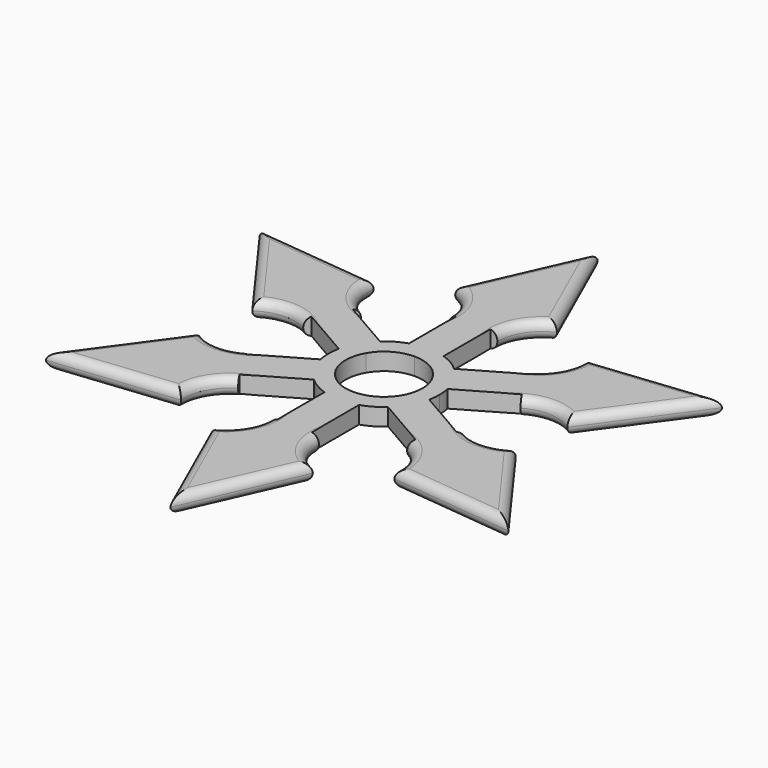
from build123d import *

# Parameters (mm, degrees)
F1_DEPTH     = 5
F2_DEPTH     = 5
F3_T1_DEPTH  = 48.744289009
F3_T3_DEPTH  = 48.744289009
F3_T5_DEPTH  = 48.744289009
F3_T7_DEPTH  = 48.744289009
F3_T9_DEPTH  = 48.744289009
F3_T11_DEPTH = 48.744289009
F3_T13_DEPTH = 48.744289009
F3_T15_DEPTH = 48.744289009
F3_T17_DEPTH = 48.744289009
F3_T19_DEPTH = 48.744289009
F3_T21_DEPTH = 48.744289009
F3_T23_DEPTH = 48.744289009
F3_T26_ANGLE = 121.141520227
F3_T28_ANGLE = 121.141520227
F3_T30_ANGLE = 121.141520227
F3_T32_ANGLE = 121.141520227
F3_T34_ANGLE = 121.141520227
F3_T36_ANGLE = 121.141520227
F3_T38_ANGLE = 121.141520227
F3_T40_ANGLE = 121.141520227
F3_T42_ANGLE = 121.141520227
F3_T44_ANGLE = 121.141520227
F3_T46_ANGLE = 121.141520227
F3_T48_ANGLE = 121.141520227
F3_T50_ANGLE = 121.141520227
F3_T52_ANGLE = 121.141520227
F3_T54_ANGLE = 121.141520227
F3_T56_ANGLE = 121.141520227
F3_T58_ANGLE = 121.141520227
F3_T60_ANGLE = 121.141520227
F3_T62_ANGLE = 121.141520227
F3_T64_ANGLE = 121.141520227
F3_T66_ANGLE = 121.141520227
F3_T68_ANGLE = 121.141520227
F3_T70_ANGLE = 121.141520227
F3_T72_ANGLE = 121.141520227


# Not quite as in the source:
# - a fillet or chamfer that OpenCascade refuses, or shapes differently, is made with other operations: its cross-section is extruded or revolved along the edge and cut away or added


with BuildPart() as f1:
    # F0 (on Top) → F1 (new body)
    with BuildSketch(Plane.XY):
        with BuildLine():
            Line((-27.9760162852, 16.1519605331), (-13.9430090009, 8.05))
            ThreePointArc((-13.9430090009, 8.05), (-12.5038298049, 10.142200955), (-10.7535844208, 11.982087552))
            Line((-10.7535844208, 11.982087552), (-25.4760162852, 20.482087552))
            Line((-25.4760162852, 20.482087552), (-27.9760162852, 16.1519605331))
        make_face()
        with BuildLine():
            ThreePointArc((-15.7535844208, 3.3218335142), (-15.0353185797, 5.7575337781), (-13.9430090009, 8.05))
            Line((-13.9430090009, 8.05), (-27.9760162852, 16.1519605331))
            Line((-27.9760162852, 16.1519605331), (-30.4760162852, 11.8218335142))
            Line((-30.4760162852, 11.8218335142), (-15.7535844208, 3.3218335142))
        make_face()
        with BuildLine():
            ThreePointArc((-9.612881982, -5.55), (-11.1, 0), (-9.612881982, 5.55))
            Line((-9.612881982, 5.55), (-13.9430090009, 8.05))
            ThreePointArc((-13.9430090009, 8.05), (-15.0353185797, 5.7575337781), (-15.7535844208, 3.3218335142))
            ThreePointArc((-15.7535844208, 3.3218335142), (-16.1, 0), (-15.7535844208, -3.3218335142))
            ThreePointArc((-15.7535844208, -3.3218335142), (-15.0353185797, -5.7575337781), (-13.9430090009, -8.05))
            Line((-13.9430090009, -8.05), (-9.612881982, -5.55))
        make_face()
        with BuildLine():
            ThreePointArc((-9.612881982, 5.55), (-5.55, 9.612881982), (0, 11.1))
            Line((0, 11.1), (0, 16.1))
            ThreePointArc((0, 16.1), (-2.5314887749, 15.8997347331), (-5, 15.3039210662))
            ThreePointArc((-5, 15.3039210662), (-8.05, 13.9430090009), (-10.7535844208, 11.982087552))
            ThreePointArc((-10.7535844208, 11.982087552), (-12.5038298049, 10.142200955), (-13.9430090009, 8.05))
            Line((-13.9430090009, 8.05), (-9.612881982, 5.55))
        make_face()
        with BuildLine():
            ThreePointArc((0, 11.1), (5.55, 9.612881982), (9.612881982, 5.55))
            Line((9.612881982, 5.55), (13.9430090009, 8.05))
            ThreePointArc((13.9430090009, 8.05), (12.5038298049, 10.142200955), (10.7535844208, 11.982087552))
            ThreePointArc((10.7535844208, 11.982087552), (8.05, 13.9430090009), (5, 15.3039210662))
            ThreePointArc((5, 15.3039210662), (2.5314887749, 15.8997347331), (0, 16.1))
            Line((0, 16.1), (0, 11.1))
        make_face()
        with BuildLine():
            ThreePointArc((9.612881982, 5.55), (10.7217766718, 2.8728914006), (11.1, 0))
            ThreePointArc((11.1, 0), (10.7217766718, -2.8728914006), (9.612881982, -5.55))
            Line((9.612881982, -5.55), (13.9430090009, -8.05))
            ThreePointArc((13.9430090009, -8.05), (15.0353185797, -5.7575337781), (15.7535844208, -3.3218335142))
            ThreePointArc((15.7535844208, -3.3218335142), (16.0131619172, -1.6699237744), (16.1, 0))
            ThreePointArc((16.1, 0), (16.0131619172, 1.6699237744), (15.7535844208, 3.3218335142))
            ThreePointArc((15.7535844208, 3.3218335142), (15.0353185797, 5.7575337781), (13.9430090009, 8.05))
            Line((13.9430090009, 8.05), (9.612881982, 5.55))
        make_face()
        with BuildLine():
            Line((13.9430090009, -8.05), (9.612881982, -5.55))
            ThreePointArc((9.612881982, -5.55), (5.55, -9.612881982), (0, -11.1))
            Line((0, -11.1), (0, -16.1))
            ThreePointArc((0, -16.1), (2.5314887749, -15.8997347331), (5, -15.3039210662))
            ThreePointArc((5, -15.3039210662), (8.05, -13.9430090009), (10.7535844208, -11.982087552))
            ThreePointArc((10.7535844208, -11.982087552), (12.5038298049, -10.142200955), (13.9430090009, -8.05))
        make_face()
        with BuildLine():
            Line((0, -16.1), (0, -11.1))
            ThreePointArc((0, -11.1), (-5.55, -9.612881982), (-9.612881982, -5.55))
            Line((-9.612881982, -5.55), (-13.9430090009, -8.05))
            ThreePointArc((-13.9430090009, -8.05), (-12.5038298049, -10.142200955), (-10.7535844208, -11.982087552))
            ThreePointArc((-10.7535844208, -11.982087552), (-8.05, -13.9430090009), (-5, -15.3039210662))
            ThreePointArc((-5, -15.3039210662), (-2.5314887749, -15.8997347331), (0, -16.1))
        make_face()
        with BuildLine():
            ThreePointArc((-10.7535844208, -11.982087552), (-12.5038298049, -10.142200955), (-13.9430090009, -8.05))
            Line((-13.9430090009, -8.05), (-27.9760162852, -16.1519605331))
            Line((-27.9760162852, -16.1519605331), (-25.4760162852, -20.482087552))
            Line((-25.4760162852, -20.482087552), (-10.7535844208, -11.982087552))
        make_face()
        with BuildLine():
            Line((-27.9760162852, -16.1519605331), (-13.9430090009, -8.05))
            ThreePointArc((-13.9430090009, -8.05), (-15.0353185797, -5.7575337781), (-15.7535844208, -3.3218335142))
            Line((-15.7535844208, -3.3218335142), (-30.4760162852, -11.8218335142))
            Line((-30.4760162852, -11.8218335142), (-27.9760162852, -16.1519605331))
        make_face()
        with BuildLine():
            ThreePointArc((10.7535844208, 11.982087552), (12.5038298049, 10.142200955), (13.9430090009, 8.05))
            Line((13.9430090009, 8.05), (27.9760162852, 16.1519605331))
            Line((27.9760162852, 16.1519605331), (25.4760162852, 20.482087552))
            Line((25.4760162852, 20.482087552), (10.7535844208, 11.982087552))
        make_face()
        with BuildLine():
            Line((27.9760162852, 16.1519605331), (13.9430090009, 8.05))
            ThreePointArc((13.9430090009, 8.05), (15.0353185797, 5.7575337781), (15.7535844208, 3.3218335142))
            Line((15.7535844208, 3.3218335142), (30.4760162852, 11.8218335142))
            Line((30.4760162852, 11.8218335142), (27.9760162852, 16.1519605331))
        make_face()
        with BuildLine():
            Line((0, 32.3039210662), (0, 16.1))
            ThreePointArc((0, 16.1), (2.5314887749, 15.8997347331), (5, 15.3039210662))
            Line((5, 15.3039210662), (5, 32.3039210662))
            Line((5, 32.3039210662), (0, 32.3039210662))
        make_face()
        with BuildLine():
            ThreePointArc((-5, 15.3039210662), (-2.5314887749, 15.8997347331), (0, 16.1))
            Line((0, 16.1), (0, 32.3039210662))
            Line((0, 32.3039210662), (-5, 32.3039210662))
            Line((-5, 32.3039210662), (-5, 15.3039210662))
        make_face()
        with BuildLine():
            ThreePointArc((15.7535844208, -3.3218335142), (15.0353185797, -5.7575337781), (13.9430090009, -8.05))
            Line((13.9430090009, -8.05), (27.9760162852, -16.1519605331))
            Line((27.9760162852, -16.1519605331), (30.4760162852, -11.8218335142))
            Line((30.4760162852, -11.8218335142), (15.7535844208, -3.3218335142))
        make_face()
        with BuildLine():
            Line((27.9760162852, -16.1519605331), (13.9430090009, -8.05))
            ThreePointArc((13.9430090009, -8.05), (12.5038298049, -10.142200955), (10.7535844208, -11.982087552))
            Line((10.7535844208, -11.982087552), (25.4760162852, -20.482087552))
            Line((25.4760162852, -20.482087552), (27.9760162852, -16.1519605331))
        make_face()
        with BuildLine():
            ThreePointArc((5, -15.3039210662), (2.5314887749, -15.8997347331), (0, -16.1))
            Line((0, -16.1), (0, -32.3039210662))
            Line((0, -32.3039210662), (5, -32.3039210662))
            Line((5, -32.3039210662), (5, -15.3039210662))
        make_face()
        with BuildLine():
            Line((0, -32.3039210662), (0, -16.1))
            ThreePointArc((0, -16.1), (-2.5314887749, -15.8997347331), (-5, -15.3039210662))
            Line((-5, -15.3039210662), (-5, -32.3039210662))
            Line((-5, -32.3039210662), (0, -32.3039210662))
        make_face()
    extrude(amount=F1_DEPTH)

    # F0 (on Top) → F2 (join)
    with BuildSketch(Plane.XY):
        with BuildLine():
            Line((-66.9471594555, 38.6519605331), (-27.9760162852, 16.1519605331))
            Line((-27.9760162852, 16.1519605331), (-25.4760162852, 20.482087552))
            Line((-25.4760162852, 20.482087552), (-24.4760162852, 22.2141383596))
            ThreePointArc((-24.4760162852, 22.2141383596), (-29.5610324314, 27.5743840984), (-30.9039085144, 34.8398026971))
            Line((-30.9039085144, 34.8398026971), (-66.9471594555, 38.6519605331))
        make_face()
        with BuildLine():
            Line((-30.4760162852, 11.8218335142), (-27.9760162852, 16.1519605331))
            Line((-27.9760162852, 16.1519605331), (-66.9471594555, 38.6519605331))
            Line((-66.9471594555, 38.6519605331), (-45.6241084557, 9.3436685012))
            ThreePointArc((-45.6241084557, 9.3436685012), (-38.6606333386, 11.8134129985), (-31.4760162852, 10.0897827066))
            Line((-31.4760162852, 10.0897827066), (-30.4760162852, 11.8218335142))
        make_face()
        with BuildLine():
            Line((-5, 32.3039210662), (0, 32.3039210662))
            Line((0, 32.3039210662), (0, 77.3039210662))
            Line((0, 77.3039210662), (-14.7201999413, 44.1834711982))
            ThreePointArc((-14.7201999413, 44.1834711982), (-9.0996009072, 39.3877970969), (-7, 32.3039210662))
            Line((-7, 32.3039210662), (-5, 32.3039210662))
        make_face()
        with BuildLine():
            Line((0, 77.3039210662), (0, 32.3039210662))
            Line((0, 32.3039210662), (5, 32.3039210662))
            Line((5, 32.3039210662), (7, 32.3039210662))
            ThreePointArc((7, 32.3039210662), (9.0996009072, 39.3877970969), (14.7201999413, 44.1834711982))
            Line((14.7201999413, 44.1834711982), (0, 77.3039210662))
        make_face()
        with BuildLine():
            Line((25.4760162852, 20.482087552), (27.9760162852, 16.1519605331))
            Line((27.9760162852, 16.1519605331), (66.9471594555, 38.6519605331))
            Line((66.9471594555, 38.6519605331), (30.9039085144, 34.8398026971))
            ThreePointArc((30.9039085144, 34.8398026971), (29.5610324314, 27.5743840984), (24.4760162852, 22.2141383596))
            Line((24.4760162852, 22.2141383596), (25.4760162852, 20.482087552))
        make_face()
        with BuildLine():
            Line((66.9471594555, 38.6519605331), (27.9760162852, 16.1519605331))
            Line((27.9760162852, 16.1519605331), (30.4760162852, 11.8218335142))
            Line((30.4760162852, 11.8218335142), (31.4760162852, 10.0897827066))
            ThreePointArc((31.4760162852, 10.0897827066), (38.6606333386, 11.8134129985), (45.6241084557, 9.3436685012))
            Line((45.6241084557, 9.3436685012), (66.9471594555, 38.6519605331))
        make_face()
        with BuildLine():
            Line((30.4760162852, -11.8218335142), (27.9760162852, -16.1519605331))
            Line((27.9760162852, -16.1519605331), (66.9471594555, -38.6519605331))
            Line((66.9471594555, -38.6519605331), (45.6241084557, -9.3436685012))
            ThreePointArc((45.6241084557, -9.3436685012), (38.6606333386, -11.8134129985), (31.4760162852, -10.0897827066))
            Line((31.4760162852, -10.0897827066), (30.4760162852, -11.8218335142))
        make_face()
        with BuildLine():
            Line((66.9471594555, -38.6519605331), (27.9760162852, -16.1519605331))
            Line((27.9760162852, -16.1519605331), (25.4760162852, -20.482087552))
            Line((25.4760162852, -20.482087552), (24.4760162852, -22.2141383596))
            ThreePointArc((24.4760162852, -22.2141383596), (29.5610324314, -27.5743840984), (30.9039085144, -34.8398026971))
            Line((30.9039085144, -34.8398026971), (66.9471594555, -38.6519605331))
        make_face()
        with BuildLine():
            Line((5, -32.3039210662), (0, -32.3039210662))
            Line((0, -32.3039210662), (0, -77.3039210662))
            Line((0, -77.3039210662), (14.7201999413, -44.1834711982))
            ThreePointArc((14.7201999413, -44.1834711982), (9.0996009072, -39.3877970969), (7, -32.3039210662))
            Line((7, -32.3039210662), (5, -32.3039210662))
        make_face()
        with BuildLine():
            Line((0, -77.3039210662), (0, -32.3039210662))
            Line((0, -32.3039210662), (-5, -32.3039210662))
            Line((-5, -32.3039210662), (-7, -32.3039210662))
            ThreePointArc((-7, -32.3039210662), (-9.0996009072, -39.3877970969), (-14.7201999413, -44.1834711982))
            Line((-14.7201999413, -44.1834711982), (0, -77.3039210662))
        make_face()
        with BuildLine():
            Line((-25.4760162852, -20.482087552), (-27.9760162852, -16.1519605331))
            Line((-27.9760162852, -16.1519605331), (-66.9471594555, -38.6519605331))
            Line((-66.9471594555, -38.6519605331), (-30.9039085144, -34.8398026971))
            ThreePointArc((-30.9039085144, -34.8398026971), (-29.5610324314, -27.5743840984), (-24.4760162852, -22.2141383596))
            Line((-24.4760162852, -22.2141383596), (-25.4760162852, -20.482087552))
        make_face()
        with BuildLine():
            Line((-66.9471594555, -38.6519605331), (-27.9760162852, -16.1519605331))
            Line((-27.9760162852, -16.1519605331), (-30.4760162852, -11.8218335142))
            Line((-30.4760162852, -11.8218335142), (-31.4760162852, -10.0897827066))
            ThreePointArc((-31.4760162852, -10.0897827066), (-38.6606333386, -11.8134129985), (-45.6241084557, -9.3436685012))
            Line((-45.6241084557, -9.3436685012), (-66.9471594555, -38.6519605331))
        make_face()
    extrude(amount=F2_DEPTH)

    # F3: fillet of radius 2.5 on 48 edges, made by hand

    # F3_s2 → F3_t1 (cut)
    with BuildSketch(Plane(origin=(-76.4647193498, -8.0873831144, 0), x_dir=(0, 0, 1), z_dir=(0.9944532484, 0.1051795453, 0))):
        with BuildLine():
            ThreePointArc((5, 28.8960959217), (4.267766953, 30.6638628747), (2.5, 31.3960959217))
            Line((2.5, 31.3960959217), (5, 31.3960959217))
            Line((5, 31.3960959217), (5, 28.8960959217))
        make_face()
        with BuildLine():
            ThreePointArc((0, 28.8960959217), (0.732233047, 30.6638628747), (2.5, 31.3960959217))
            Line((2.5, 31.3960959217), (0, 31.3960959217))
            Line((0, 31.3960959217), (0, 28.8960959217))
        make_face()
    extrude(amount=F3_T1_DEPTH, mode=Mode.SUBTRACT)

    # F3_s4 → F3_t3 (cut)
    with BuildSketch(Plane(origin=(-16.5592531229, -22.760505819, 0), x_dir=(0, 0, 1), z_dir=(-0.5883147824, -0.8086320034, 0))):
        with BuildLine():
            ThreePointArc((5, 28.8960959217), (4.267766953, 30.6638628747), (2.5, 31.3960959217))
            Line((2.5, 31.3960959217), (5, 31.3960959217))
            Line((5, 31.3960959217), (5, 28.8960959217))
        make_face()
        with BuildLine():
            ThreePointArc((0, 28.8960959217), (0.732233047, 30.6638628747), (2.5, 31.3960959217))
            Line((2.5, 31.3960959217), (0, 31.3960959217))
            Line((0, 31.3960959217), (0, 28.8960959217))
        make_face()
    extrude(amount=F3_T3_DEPTH, mode=Mode.SUBTRACT)

    # F3_s6 → F3_t5 (cut)
    with BuildSketch(Plane(origin=(11.4315496807, -25.7209867816, 0), x_dir=(0, 0, 1), z_dir=(0.4061384661, -0.9138115486, 0))):
        with BuildLine():
            ThreePointArc((5, 28.8960959217), (4.267766953, 30.6638628747), (2.5, 31.3960959217))
            Line((2.5, 31.3960959217), (5, 31.3960959217))
            Line((5, 31.3960959217), (5, 28.8960959217))
        make_face()
        with BuildLine():
            ThreePointArc((0, 28.8960959217), (0.732233047, 30.6638628747), (2.5, 31.3960959217))
            Line((2.5, 31.3960959217), (0, 31.3960959217))
            Line((0, 31.3960959217), (0, 28.8960959217))
        make_face()
    extrude(amount=F3_T5_DEPTH, mode=Mode.SUBTRACT)

    # F3_s8 → F3_t7 (cut)
    with BuildSketch(Plane(origin=(-31.2284804477, -70.2640810073, 0), x_dir=(0, 0, 1), z_dir=(0.4061384661, 0.9138115486, 0))):
        with BuildLine():
            ThreePointArc((5, 28.8960959217), (4.267766953, 30.6638628747), (2.5, 31.3960959217))
            Line((2.5, 31.3960959217), (5, 31.3960959217))
            Line((5, 31.3960959217), (5, 28.8960959217))
        make_face()
        with BuildLine():
            ThreePointArc((0, 28.8960959217), (0.732233047, 30.6638628747), (2.5, 31.3960959217))
            Line((2.5, 31.3960959217), (0, 31.3960959217))
            Line((0, 31.3960959217), (0, 28.8960959217))
        make_face()
    extrude(amount=F3_T7_DEPTH, mode=Mode.SUBTRACT)

    # F3_s10 → F3_t9 (cut)
    with BuildSketch(Plane(origin=(45.2362389021, -62.176697893, 0), x_dir=(0, 0, 1), z_dir=(-0.5883147824, 0.8086320034, 0))):
        with BuildLine():
            ThreePointArc((5, 28.8960959217), (4.267766953, 30.6638628747), (2.5, 31.3960959217))
            Line((2.5, 31.3960959217), (5, 31.3960959217))
            Line((5, 31.3960959217), (5, 28.8960959217))
        make_face()
        with BuildLine():
            ThreePointArc((0, 28.8960959217), (0.732233047, 30.6638628747), (2.5, 31.3960959217))
            Line((2.5, 31.3960959217), (0, 31.3960959217))
            Line((0, 31.3960959217), (0, 28.8960959217))
        make_face()
    extrude(amount=F3_T9_DEPTH, mode=Mode.SUBTRACT)

    # F3_s12 → F3_t11 (cut)
    with BuildSketch(Plane(origin=(27.9908028037, -2.9604809627, 0), x_dir=(0, 0, 1), z_dir=(0.9944532484, -0.1051795453, 0))):
        with BuildLine():
            ThreePointArc((5, 28.8960959217), (4.267766953, 30.6638628747), (2.5, 31.3960959217))
            Line((2.5, 31.3960959217), (5, 31.3960959217))
            Line((5, 31.3960959217), (5, 28.8960959217))
        make_face()
        with BuildLine():
            ThreePointArc((0, 28.8960959217), (0.732233047, 30.6638628747), (2.5, 31.3960959217))
            Line((2.5, 31.3960959217), (0, 31.3960959217))
            Line((0, 31.3960959217), (0, 28.8960959217))
        make_face()
    extrude(amount=F3_T11_DEPTH, mode=Mode.SUBTRACT)

    # F3_s14 → F3_t13 (cut)
    with BuildSketch(Plane(origin=(76.4647193498, 8.0873831144, 0), x_dir=(0, 0, 1), z_dir=(-0.9944532484, -0.1051795453, 0))):
        with BuildLine():
            ThreePointArc((5, 28.8960959217), (4.267766953, 30.6638628747), (2.5, 31.3960959217))
            Line((2.5, 31.3960959217), (5, 31.3960959217))
            Line((5, 31.3960959217), (5, 28.8960959217))
        make_face()
        with BuildLine():
            ThreePointArc((0, 28.8960959217), (0.732233047, 30.6638628747), (2.5, 31.3960959217))
            Line((2.5, 31.3960959217), (0, 31.3960959217))
            Line((0, 31.3960959217), (0, 28.8960959217))
        make_face()
    extrude(amount=F3_T13_DEPTH, mode=Mode.SUBTRACT)

    # F3_s16 → F3_t15 (cut)
    with BuildSketch(Plane(origin=(16.5592531229, 22.760505819, 0), x_dir=(0, 0, 1), z_dir=(0.5883147824, 0.8086320034, 0))):
        with BuildLine():
            ThreePointArc((5, 28.8960959217), (4.267766953, 30.6638628747), (2.5, 31.3960959217))
            Line((2.5, 31.3960959217), (5, 31.3960959217))
            Line((5, 31.3960959217), (5, 28.8960959217))
        make_face()
        with BuildLine():
            ThreePointArc((0, 28.8960959217), (0.732233047, 30.6638628747), (2.5, 31.3960959217))
            Line((2.5, 31.3960959217), (0, 31.3960959217))
            Line((0, 31.3960959217), (0, 28.8960959217))
        make_face()
    extrude(amount=F3_T15_DEPTH, mode=Mode.SUBTRACT)

    # F3_s18 → F3_t17 (cut)
    with BuildSketch(Plane(origin=(-27.9908028037, 2.9604809627, 0), x_dir=(0, 0, 1), z_dir=(-0.9944532484, 0.1051795453, 0))):
        with BuildLine():
            ThreePointArc((2.5, 31.3960959217), (4.267766953, 30.6638628747), (5, 28.8960959217))
            Line((5, 28.8960959217), (5, 31.3960959217))
            Line((5, 31.3960959217), (2.5, 31.3960959217))
        make_face()
        with BuildLine():
            ThreePointArc((2.5, 31.3960959217), (0.732233047, 30.6638628747), (0, 28.8960959217))
            Line((0, 28.8960959217), (0, 31.3960959217))
            Line((0, 31.3960959217), (2.5, 31.3960959217))
        make_face()
    extrude(amount=F3_T17_DEPTH, mode=Mode.SUBTRACT)

    # F3_s20 → F3_t19 (cut)
    with BuildSketch(Plane(origin=(-45.2362389021, 62.176697893, 0), x_dir=(0, 0, 1), z_dir=(0.5883147824, -0.8086320034, 0))):
        with BuildLine():
            ThreePointArc((2.5, 31.3960959217), (4.267766953, 30.6638628747), (5, 28.8960959217))
            Line((5, 28.8960959217), (5, 31.3960959217))
            Line((5, 31.3960959217), (2.5, 31.3960959217))
        make_face()
        with BuildLine():
            ThreePointArc((2.5, 31.3960959217), (0.732233047, 30.6638628747), (0, 28.8960959217))
            Line((0, 28.8960959217), (0, 31.3960959217))
            Line((0, 31.3960959217), (2.5, 31.3960959217))
        make_face()
    extrude(amount=F3_T19_DEPTH, mode=Mode.SUBTRACT)

    # F3_s22 → F3_t21 (cut)
    with BuildSketch(Plane(origin=(31.2284804477, 70.2640810073, 0), x_dir=(0, 0, 1), z_dir=(-0.4061384661, -0.9138115486, 0))):
        with BuildLine():
            ThreePointArc((5, 28.8960959217), (4.267766953, 30.6638628747), (2.5, 31.3960959217))
            Line((2.5, 31.3960959217), (5, 31.3960959217))
            Line((5, 31.3960959217), (5, 28.8960959217))
        make_face()
        with BuildLine():
            ThreePointArc((0, 28.8960959217), (0.732233047, 30.6638628747), (2.5, 31.3960959217))
            Line((2.5, 31.3960959217), (0, 31.3960959217))
            Line((0, 31.3960959217), (0, 28.8960959217))
        make_face()
    extrude(amount=F3_T21_DEPTH, mode=Mode.SUBTRACT)

    # F3_s24 → F3_t23 (cut)
    with BuildSketch(Plane(origin=(-11.4315496807, 25.7209867816, 0), x_dir=(0, 0, 1), z_dir=(-0.4061384661, 0.9138115486, 0))):
        with BuildLine():
            ThreePointArc((5, 28.8960959217), (4.267766953, 30.6638628747), (2.5, 31.3960959217))
            Line((2.5, 31.3960959217), (5, 31.3960959217))
            Line((5, 31.3960959217), (5, 28.8960959217))
        make_face()
        with BuildLine():
            ThreePointArc((0, 28.8960959217), (0.732233047, 30.6638628747), (2.5, 31.3960959217))
            Line((2.5, 31.3960959217), (0, 31.3960959217))
            Line((0, 31.3960959217), (0, 28.8960959217))
        make_face()
    extrude(amount=F3_T23_DEPTH, mode=Mode.SUBTRACT)

    # F3_s25 → F3_t26 (revolve, cut)
    with BuildSketch(Plane(origin=(19.3716122948, -0.8281673611, 0), x_dir=(0, 0, 1), z_dir=(-0.9990874013, 0.0427125819, 0))):
        with BuildLine():
            ThreePointArc((0, -17.1741196082), (0.732233047, -18.9418865612), (2.5, -19.6741196082))
            Line((2.5, -19.6741196082), (0, -19.6741196082))
            Line((0, -19.6741196082), (0, -17.1741196082))
        make_face()
    revolve(axis=Axis((17.9760162852, -33.4724686088, 0), (0, 0, -1)), revolution_arc=F3_T26_ANGLE, mode=Mode.SUBTRACT)

    # F3_s27 → F3_t28 (revolve, cut)
    with BuildSketch(Plane(origin=(19.3716122948, -0.8281673611, 0), x_dir=(0, 0, 1), z_dir=(-0.9990874013, 0.0427125819, 0))):
        with BuildLine():
            ThreePointArc((5, -17.1741196082), (4.267766953, -18.9418865612), (2.5, -19.6741196082))
            Line((2.5, -19.6741196082), (5, -19.6741196082))
            Line((5, -19.6741196082), (5, -17.1741196082))
        make_face()
    revolve(axis=Axis((17.9760162852, -33.4724686088, 5), (0, 0, -1)), revolution_arc=F3_T28_ANGLE, mode=Mode.SUBTRACT)

    # F3_s29 → F3_t30 (revolve, cut)
    with BuildSketch(Plane(origin=(7.978931959, 16.0660718144, 0), x_dir=(0, 0, 1), z_dir=(0.4447990752, 0.8956303829, 0))):
        with BuildLine():
            ThreePointArc((0, 48.9927051385), (0.732233047, 47.2249381856), (2.5, 46.4927051385))
            Line((2.5, 46.4927051385), (0, 46.4927051385))
            Line((0, 46.4927051385), (0, 48.9927051385))
        make_face()
    revolve(axis=Axis((37.9760162852, 1.1685475426, 0), (0, 0, -1)), revolution_arc=F3_T30_ANGLE, mode=Mode.SUBTRACT)

    # F3_s31 → F3_t32 (revolve, cut)
    with BuildSketch(Plane(origin=(7.978931959, 16.0660718144, 0), x_dir=(0, 0, 1), z_dir=(0.4447990752, 0.8956303829, 0))):
        with BuildLine():
            ThreePointArc((5, 48.9927051385), (4.267766953, 47.2249381856), (2.5, 46.4927051385))
            Line((2.5, 46.4927051385), (5, 46.4927051385))
            Line((5, 46.4927051385), (5, 48.9927051385))
        make_face()
    revolve(axis=Axis((37.9760162852, 1.1685475426, 5), (0, 0, -1)), revolution_arc=F3_T32_ANGLE, mode=Mode.SUBTRACT)

    # F3_s33 → F3_t34 (revolve, cut)
    with BuildSketch(Plane(origin=(10.4030201207, 16.362224679, 0), x_dir=(0, 0, 1), z_dir=(-0.5365338816, -0.8438787791, 0))):
        with BuildLine():
            ThreePointArc((5, -17.1741196082), (4.267766953, -18.9418865612), (2.5, -19.6741196082))
            Line((2.5, -19.6741196082), (5, -19.6741196082))
            Line((5, -19.6741196082), (5, -17.1741196082))
        make_face()
    revolve(axis=Axis((37.9760162852, -1.1685475426, 5), (0, 0, -1)), revolution_arc=F3_T34_ANGLE, mode=Mode.SUBTRACT)

    # F3_s35 → F3_t36 (revolve, cut)
    with BuildSketch(Plane(origin=(10.4030201207, 16.362224679, 0), x_dir=(0, 0, 1), z_dir=(-0.5365338816, -0.8438787791, 0))):
        with BuildLine():
            ThreePointArc((0, -17.1741196082), (0.732233047, -18.9418865612), (2.5, -19.6741196082))
            Line((2.5, -19.6741196082), (0, -19.6741196082))
            Line((0, -19.6741196082), (0, -17.1741196082))
        make_face()
    revolve(axis=Axis((37.9760162852, -1.1685475426, 0), (0, 0, -1)), revolution_arc=F3_T36_ANGLE, mode=Mode.SUBTRACT)

    # F3_s37 → F3_t38 (revolve, cut)
    with BuildSketch(Plane(origin=(-9.9241603508, 14.9429936788, 0), x_dir=(0, 0, 1), z_dir=(-0.5532391264, 0.8330224901, 0))):
        with BuildLine():
            ThreePointArc((5, 48.9927051385), (4.267766953, 47.2249381856), (2.5, 46.4927051385))
            Line((2.5, 46.4927051385), (5, 46.4927051385))
            Line((5, 46.4927051385), (5, 48.9927051385))
        make_face()
    revolve(axis=Axis((17.9760162852, 33.4724686088, 5), (0, 0, -1)), revolution_arc=F3_T38_ANGLE, mode=Mode.SUBTRACT)

    # F3_s39 → F3_t40 (revolve, cut)
    with BuildSketch(Plane(origin=(-9.9241603508, 14.9429936788, 0), x_dir=(0, 0, 1), z_dir=(-0.5532391264, 0.8330224901, 0))):
        with BuildLine():
            ThreePointArc((0, 48.9927051385), (0.732233047, 47.2249381856), (2.5, 46.4927051385))
            Line((2.5, 46.4927051385), (0, 46.4927051385))
            Line((0, 46.4927051385), (0, 48.9927051385))
        make_face()
    revolve(axis=Axis((17.9760162852, 33.4724686088, 0), (0, 0, -1)), revolution_arc=F3_T40_ANGLE, mode=Mode.SUBTRACT)

    # F3_s41 → F3_t42 (revolve, cut)
    with BuildSketch(Plane(origin=(-8.9685921741, 17.1903920401, 0), x_dir=(0, 0, 1), z_dir=(0.4625535196, -0.886591361, 0))):
        with BuildLine():
            ThreePointArc((5, -17.1741196082), (4.267766953, -18.9418865612), (2.5, -19.6741196082))
            Line((2.5, -19.6741196082), (5, -19.6741196082))
            Line((5, -19.6741196082), (5, -17.1741196082))
        make_face()
    revolve(axis=Axis((20, 32.3039210662, 5), (0, 0, -1)), revolution_arc=F3_T42_ANGLE, mode=Mode.SUBTRACT)

    # F3_s43 → F3_t44 (revolve, cut)
    with BuildSketch(Plane(origin=(-8.9685921741, 17.1903920401, 0), x_dir=(0, 0, 1), z_dir=(0.4625535196, -0.886591361, 0))):
        with BuildLine():
            ThreePointArc((0, -17.1741196082), (0.732233047, -18.9418865612), (2.5, -19.6741196082))
            Line((2.5, -19.6741196082), (0, -19.6741196082))
            Line((0, -19.6741196082), (0, -17.1741196082))
        make_face()
    revolve(axis=Axis((20, 32.3039210662, 0), (0, 0, -1)), revolution_arc=F3_T44_ANGLE, mode=Mode.SUBTRACT)

    # F3_s45 → F3_t46 (revolve, cut)
    with BuildSketch(Plane(origin=(-17.9030923098, -1.1230781356, 0), x_dir=(0, 0, 1), z_dir=(-0.9980382016, -0.0626078927, 0))):
        with BuildLine():
            ThreePointArc((0, 48.9927051385), (0.732233047, 47.2249381856), (2.5, 46.4927051385))
            Line((2.5, 46.4927051385), (0, 46.4927051385))
            Line((0, 46.4927051385), (0, 48.9927051385))
        make_face()
    revolve(axis=Axis((-20, 32.3039210662, 0), (0, 0, -1)), revolution_arc=F3_T46_ANGLE, mode=Mode.SUBTRACT)

    # F3_s47 → F3_t48 (revolve, cut)
    with BuildSketch(Plane(origin=(-17.9030923098, -1.1230781356, 0), x_dir=(0, 0, 1), z_dir=(-0.9980382016, -0.0626078927, 0))):
        with BuildLine():
            ThreePointArc((5, 48.9927051385), (4.267766953, 47.2249381856), (2.5, 46.4927051385))
            Line((2.5, 46.4927051385), (5, 46.4927051385))
            Line((5, 46.4927051385), (5, 48.9927051385))
        make_face()
    revolve(axis=Axis((-20, 32.3039210662, 5), (0, 0, -1)), revolution_arc=F3_T48_ANGLE, mode=Mode.SUBTRACT)

    # F3_s49 → F3_t50 (revolve, cut)
    with BuildSketch(Plane(origin=(-19.3716122948, 0.8281673611, 0), x_dir=(0, 0, 1), z_dir=(0.9990874013, -0.0427125819, 0))):
        with BuildLine():
            ThreePointArc((2.5, -19.6741196082), (0.732233047, -18.9418865612), (0, -17.1741196082))
            Line((0, -17.1741196082), (0, -19.6741196082))
            Line((0, -19.6741196082), (2.5, -19.6741196082))
        make_face()
    revolve(axis=Axis((-17.9760162852, 33.4724686088, 0), (0, 0, -1)), revolution_arc=F3_T50_ANGLE, mode=Mode.SUBTRACT)

    # F3_s51 → F3_t52 (revolve, cut)
    with BuildSketch(Plane(origin=(-19.3716122948, 0.8281673611, 0), x_dir=(0, 0, 1), z_dir=(0.9990874013, -0.0427125819, 0))):
        with BuildLine():
            ThreePointArc((2.5, -19.6741196082), (4.267766953, -18.9418865612), (5, -17.1741196082))
            Line((5, -17.1741196082), (5, -19.6741196082))
            Line((5, -19.6741196082), (2.5, -19.6741196082))
        make_face()
    revolve(axis=Axis((-17.9760162852, 33.4724686088, 5), (0, 0, -1)), revolution_arc=F3_T52_ANGLE, mode=Mode.SUBTRACT)

    # F3_s53 → F3_t54 (revolve, cut)
    with BuildSketch(Plane(origin=(-7.978931959, -16.0660718144, 0), x_dir=(0, 0, 1), z_dir=(-0.4447990752, -0.8956303829, 0))):
        with BuildLine():
            ThreePointArc((5, 48.9927051385), (4.267766953, 47.2249381856), (2.5, 46.4927051385))
            Line((2.5, 46.4927051385), (5, 46.4927051385))
            Line((5, 46.4927051385), (5, 48.9927051385))
        make_face()
    revolve(axis=Axis((-37.9760162852, -1.1685475426, 5), (0, 0, -1)), revolution_arc=F3_T54_ANGLE, mode=Mode.SUBTRACT)

    # F3_s55 → F3_t56 (revolve, cut)
    with BuildSketch(Plane(origin=(-7.978931959, -16.0660718144, 0), x_dir=(0, 0, 1), z_dir=(-0.4447990752, -0.8956303829, 0))):
        with BuildLine():
            ThreePointArc((0, 48.9927051385), (0.732233047, 47.2249381856), (2.5, 46.4927051385))
            Line((2.5, 46.4927051385), (0, 46.4927051385))
            Line((0, 46.4927051385), (0, 48.9927051385))
        make_face()
    revolve(axis=Axis((-37.9760162852, -1.1685475426, 0), (0, 0, -1)), revolution_arc=F3_T56_ANGLE, mode=Mode.SUBTRACT)

    # F3_s57 → F3_t58 (revolve, cut)
    with BuildSketch(Plane(origin=(-10.4030201207, -16.362224679, 0), x_dir=(0, 0, 1), z_dir=(0.5365338816, 0.8438787791, 0))):
        with BuildLine():
            ThreePointArc((5, -17.1741196082), (4.267766953, -18.9418865612), (2.5, -19.6741196082))
            Line((2.5, -19.6741196082), (5, -19.6741196082))
            Line((5, -19.6741196082), (5, -17.1741196082))
        make_face()
    revolve(axis=Axis((-37.9760162852, 1.1685475426, 5), (0, 0, -1)), revolution_arc=F3_T58_ANGLE, mode=Mode.SUBTRACT)

    # F3_s59 → F3_t60 (revolve, cut)
    with BuildSketch(Plane(origin=(-10.4030201207, -16.362224679, 0), x_dir=(0, 0, 1), z_dir=(0.5365338816, 0.8438787791, 0))):
        with BuildLine():
            ThreePointArc((0, -17.1741196082), (0.732233047, -18.9418865612), (2.5, -19.6741196082))
            Line((2.5, -19.6741196082), (0, -19.6741196082))
            Line((0, -19.6741196082), (0, -17.1741196082))
        make_face()
    revolve(axis=Axis((-37.9760162852, 1.1685475426, 0), (0, 0, -1)), revolution_arc=F3_T60_ANGLE, mode=Mode.SUBTRACT)

    # F3_s61 → F3_t62 (revolve, cut)
    with BuildSketch(Plane(origin=(9.9241603508, -14.9429936788, 0), x_dir=(0, 0, 1), z_dir=(0.5532391264, -0.8330224901, 0))):
        with BuildLine():
            ThreePointArc((5, 48.9927051385), (4.267766953, 47.2249381856), (2.5, 46.4927051385))
            Line((2.5, 46.4927051385), (5, 46.4927051385))
            Line((5, 46.4927051385), (5, 48.9927051385))
        make_face()
    revolve(axis=Axis((-17.9760162852, -33.4724686088, 5), (0, 0, -1)), revolution_arc=F3_T62_ANGLE, mode=Mode.SUBTRACT)

    # F3_s63 → F3_t64 (revolve, cut)
    with BuildSketch(Plane(origin=(9.9241603508, -14.9429936788, 0), x_dir=(0, 0, 1), z_dir=(0.5532391264, -0.8330224901, 0))):
        with BuildLine():
            ThreePointArc((0, 48.9927051385), (0.732233047, 47.2249381856), (2.5, 46.4927051385))
            Line((2.5, 46.4927051385), (0, 46.4927051385))
            Line((0, 46.4927051385), (0, 48.9927051385))
        make_face()
    revolve(axis=Axis((-17.9760162852, -33.4724686088, 0), (0, 0, -1)), revolution_arc=F3_T64_ANGLE, mode=Mode.SUBTRACT)

    # F3_s65 → F3_t66 (revolve, cut)
    with BuildSketch(Plane(origin=(17.9030923098, 1.1230781356, 0), x_dir=(0, 0, 1), z_dir=(0.9980382016, 0.0626078927, 0))):
        with BuildLine():
            ThreePointArc((5, 48.9927051385), (4.267766953, 47.2249381856), (2.5, 46.4927051385))
            Line((2.5, 46.4927051385), (5, 46.4927051385))
            Line((5, 46.4927051385), (5, 48.9927051385))
        make_face()
    revolve(axis=Axis((20, -32.3039210662, 5), (0, 0, -1)), revolution_arc=F3_T66_ANGLE, mode=Mode.SUBTRACT)

    # F3_s67 → F3_t68 (revolve, cut)
    with BuildSketch(Plane(origin=(17.9030923098, 1.1230781356, 0), x_dir=(0, 0, 1), z_dir=(0.9980382016, 0.0626078927, 0))):
        with BuildLine():
            ThreePointArc((0, 48.9927051385), (0.732233047, 47.2249381856), (2.5, 46.4927051385))
            Line((2.5, 46.4927051385), (0, 46.4927051385))
            Line((0, 46.4927051385), (0, 48.9927051385))
        make_face()
    revolve(axis=Axis((20, -32.3039210662, 0), (0, 0, -1)), revolution_arc=F3_T68_ANGLE, mode=Mode.SUBTRACT)

    # F3_s69 → F3_t70 (revolve, cut)
    with BuildSketch(Plane(origin=(8.9685921741, -17.1903920401, 0), x_dir=(0, 0, 1), z_dir=(-0.4625535196, 0.886591361, 0))):
        with BuildLine():
            ThreePointArc((5, -17.1741196082), (4.267766953, -18.9418865612), (2.5, -19.6741196082))
            Line((2.5, -19.6741196082), (5, -19.6741196082))
            Line((5, -19.6741196082), (5, -17.1741196082))
        make_face()
    revolve(axis=Axis((-20, -32.3039210662, 5), (0, 0, -1)), revolution_arc=F3_T70_ANGLE, mode=Mode.SUBTRACT)

    # F3_s71 → F3_t72 (revolve, cut)
    with BuildSketch(Plane(origin=(8.9685921741, -17.1903920401, 0), x_dir=(0, 0, 1), z_dir=(-0.4625535196, 0.886591361, 0))):
        with BuildLine():
            ThreePointArc((0, -17.1741196082), (0.732233047, -18.9418865612), (2.5, -19.6741196082))
            Line((2.5, -19.6741196082), (0, -19.6741196082))
            Line((0, -19.6741196082), (0, -17.1741196082))
        make_face()
    revolve(axis=Axis((-20, -32.3039210662, 0), (0, 0, -1)), revolution_arc=F3_T72_ANGLE, mode=Mode.SUBTRACT)


solid = f1.part
